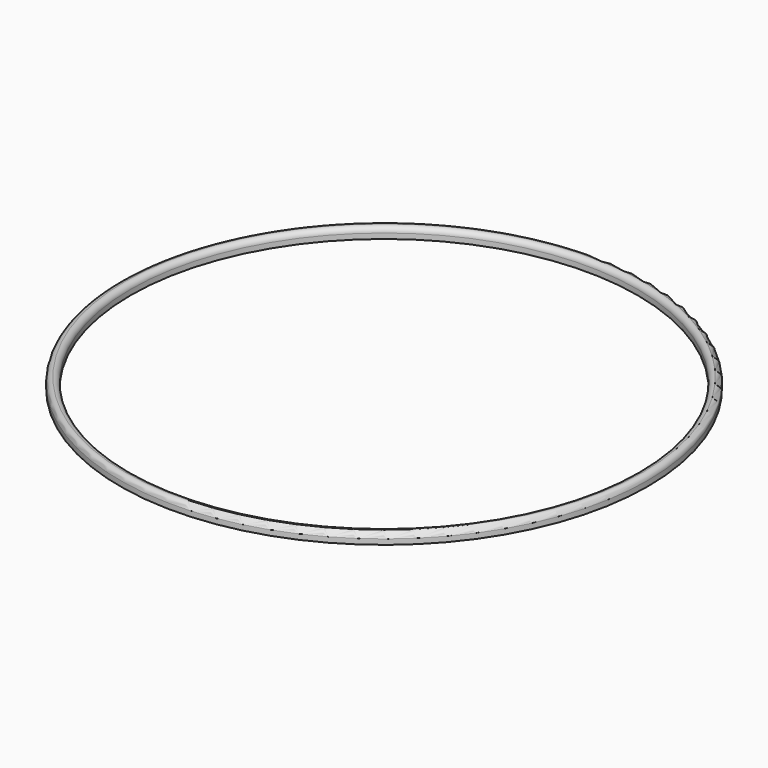
from build123d import *

# Parameters (mm, degrees)
F0_R     = 79.375
F0_R_2   = 76.2
F1_DEPTH = 3.175
F2_R     = 1.58749


# Not quite as in the source:
# - a fillet or chamfer is up to 0.001 mm smaller than in the source, because OpenCascade refuses the exact size


with BuildPart() as f1:
    # F0 (on Top) → F1 (new body)
    with BuildSketch(Plane.XY):
        Circle(F0_R)
        Circle(F0_R_2, mode=Mode.SUBTRACT)
    extrude(amount=F1_DEPTH)

    # F2 (radius 1.5875 in the source; OpenCascade refuses exactly that, so slightly less here)
    f2_edges = [f1.edges().sort_by_distance(p)[0] for p in [
        (-76.2, 0, 3.175),
        (-79.375, 0, 3.175),
    ]]
    fillet(f2_edges, radius=F2_R)


solid = f1.part
